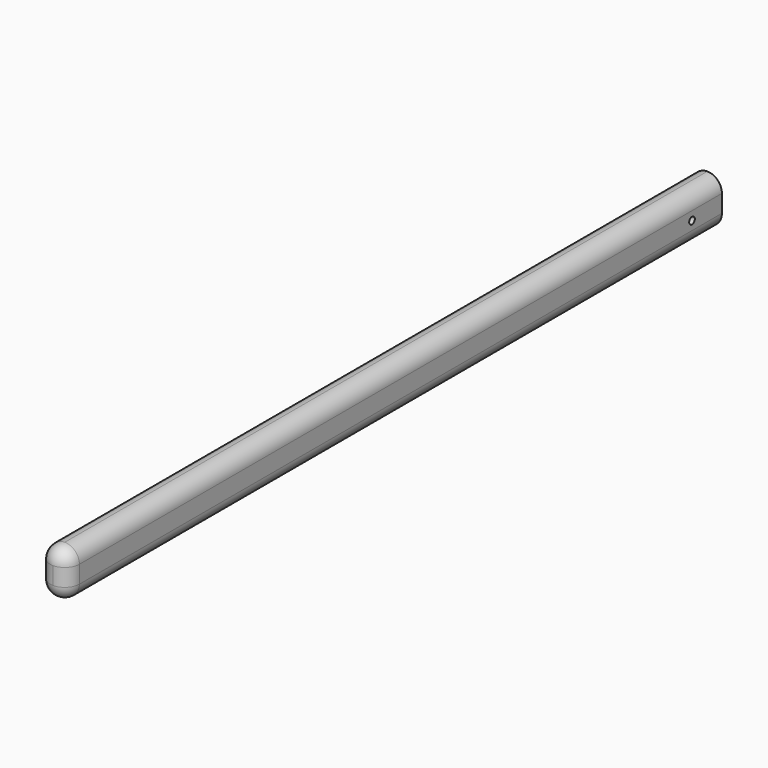
from build123d import *

# Parameters (mm, degrees)
F1_DEPTH    = 700
F2_T1_DEPTH = 15
F2_T4_ANGLE = 180
F2_T6_ANGLE = 180
F3_R        = 3
F4_DEPTH    = 25.001


# Not quite as in the source:
# - a fillet or chamfer that OpenCascade refuses, or shapes differently, is made with other operations: its cross-section is extruded or revolved along the edge and cut away or added


with BuildPart() as f1:
    # F0 (on Front) → F1 (new body)
    with BuildSketch(Plane.XZ):
        with BuildLine():
            Line((12.5, -7.5), (12.5, 7.5))
            ThreePointArc((12.5, 7.5), (8.8388347648, 16.3388347648), (0, 20))
            ThreePointArc((0, 20), (-8.8388347648, 16.3388347648), (-12.5, 7.5))
            Line((-12.5, 7.5), (-12.5, -7.5))
            ThreePointArc((-12.5, -7.5), (-8.8388347648, -16.3388347648), (0, -20))
            ThreePointArc((0, -20), (8.8388347648, -16.3388347648), (12.5, -7.5))
        make_face()
    extrude(amount=F1_DEPTH)

    # F2: fillet of radius 12.5 on 4 edges, made by hand

    # F2_s2 → F2_t1 (cut)
    with BuildSketch(Plane.XY.offset(-7.5)):
        with BuildLine():
            ThreePointArc((12.5, -687.5), (8.8388347648, -696.3388347648), (0, -700))
            Line((0, -700), (12.5, -700))
            Line((12.5, -700), (12.5, -687.5))
        make_face()
        with BuildLine():
            ThreePointArc((0, -700), (-8.8388347648, -696.3388347648), (-12.5, -687.5))
            Line((-12.5, -687.5), (-12.5, -700))
            Line((-12.5, -700), (0, -700))
        make_face()
    extrude(amount=F2_T1_DEPTH, mode=Mode.SUBTRACT)

    # F2_s3 → F2_t4 (revolve, cut)
    with BuildSketch(Plane.XY.offset(-7.5)):
        with BuildLine():
            ThreePointArc((0, -700), (8.8388347648, -696.3388347648), (12.5, -687.5))
            Line((12.5, -687.5), (12.5, -700))
            Line((12.5, -700), (0, -700))
        make_face()
    revolve(axis=Axis((0, -700, -7.5), (0, 1, 0)), revolution_arc=F2_T4_ANGLE, mode=Mode.SUBTRACT)

    # F2_s5 → F2_t6 (revolve, cut)
    with BuildSketch(Plane.XY.offset(7.5)):
        with BuildLine():
            ThreePointArc((0, -700), (-8.8388347648, -696.3388347648), (-12.5, -687.5))
            Line((-12.5, -687.5), (-12.5, -700))
            Line((-12.5, -700), (0, -700))
        make_face()
    revolve(axis=Axis((0, -700, 7.5), (0, 1, 0)), revolution_arc=F2_T6_ANGLE, mode=Mode.SUBTRACT)

    # F3 (on face) → F4 (cut, through all)
    with BuildSketch(Plane(origin=(-12.5, 0, 0), x_dir=(0, -1, 0), z_dir=(-1, 0, 0))):
        with Locations((32, 0)):
            Circle(F3_R)
    extrude(amount=-F4_DEPTH, mode=Mode.SUBTRACT)


solid = f1.part
